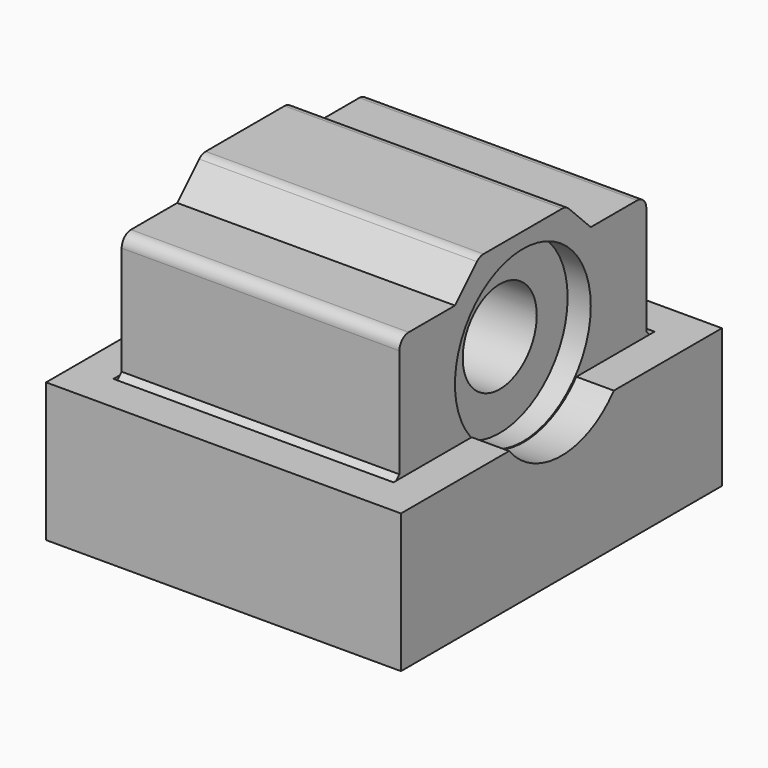
from build123d import *

# Parameters (mm, degrees)
F1_R              = 11
F2_DEPTH          = 18
F1_R_2            = 6
F3_DEPTH          = 15
F4_SIZE           = 0.99999
F5_R              = 1.5
F6_W              = 46
F6_H              = 52
F6_W_2            = 36.3
F6_H_2            = 42.3
F6_W_3            = 26
F6_H_3            = 23.35
F6_H_4            = 7.15
F7_DEPTH          = 10
F8_DEPTH          = 8
F10_D             = 5.5
F10_DEPTH         = 20
F10_CBORE_D       = 9.75
F10_CBORE_DEPTH   = 5
F10_TIP           = 1.6523667023
F10_2_D           = 5.5
F10_2_DEPTH       = 20
F10_2_CBORE_D     = 9.75
F10_2_CBORE_DEPTH = 5
F10_2_TIP         = 1.6523667023
F11_DEPTH         = 57.8


# Not quite as in the source:
# - a fillet or chamfer is up to 0.001 mm smaller than in the source, because OpenCascade refuses the exact size


with BuildPart() as f2:
    # F1 (on Right) → F2 (new body, symmetric)
    with BuildSketch(Plane.YZ):
        Polygon((-7.5, 0), (0, 0), (7.5, 0), (7.5, -1), (21, -1), (21, 6.4), (20, 6.4), (20, 23), (11, 23), (7, 27), (0, 27), (-7, 27), (-11, 23), (-20, 23), (-20, 6.4), (-21, 6.4), (-21, -1), (-7.5, -1), align=None)
        with Locations((0, 14)):
            Circle(F1_R, mode=Mode.SUBTRACT)
    extrude(amount=F2_DEPTH, both=True)

    # F4 (size 1 in the source; OpenCascade refuses exactly that, so slightly less here)
    f4_edges = [f2.edges().sort_by_distance(p)[0] for p in [
        (0, -20, 6.4),
        (0, 20, 6.4),
        (0, -7.5, 0),
        (0, 7.5, 0),
    ]]
    chamfer(f4_edges, length=F4_SIZE)

    # F5
    f5_edges = [f2.edges().sort_by_distance(p)[0] for p in [
        (0, -7, 27),
        (0, 7, 27),
        (0, -20, 23),
        (0, 20, 23),
    ]]
    fillet(f5_edges, radius=F5_R)

    # F10
    with Locations(Plane(origin=(0, 0, -11), x_dir=(1, 0, 0), z_dir=(0, 0, -1))):
        with Locations((-13, -15.85), (13, -15.85), (-13, 14.65), (13, 14.65)):
            CounterBoreHole(F10_D / 2, F10_CBORE_D / 2, F10_CBORE_DEPTH, depth=F10_DEPTH)
            with Locations((0, 0, -(F10_DEPTH + F10_TIP / 2))):  # 118° drill point
                Cone(0, F10_D / 2, F10_TIP, mode=Mode.SUBTRACT)


with BuildPart() as f3:
    # F1 (on Right) → F3 (new body, symmetric)
    with BuildSketch(Plane.YZ):
        with Locations((0, 14)):
            Circle(F1_R)
        with Locations((0, 14)):
            Circle(F1_R_2, mode=Mode.SUBTRACT)
    extrude(amount=F3_DEPTH, both=True)


with BuildPart() as f7:
    # F6 (on face) → F7 (new body)
    with BuildSketch(Plane(origin=(0, 0, -1), x_dir=(1, 0, 0), z_dir=(0, 0, -1))):
        Rectangle(F6_W, F6_H)
        Rectangle(F6_W_2, F6_H_2, mode=Mode.SUBTRACT)
        Rectangle(F6_W_2, F6_H_2)
        Polygon((18, 21), (18, 7.5), (18, -21), (-18, -21), (-18, 7.5), (-18, 21), align=None, mode=Mode.SUBTRACT)
        with Locations((0, -4.175)):
            Rectangle(F6_W_3, F6_H_3)
        Polygon((18, 7.5), (13, 7.5), (13, -15.85), (-13, -15.85), (-13, 7.5), (-18, 7.5), (-18, -21), (18, -21), align=None)
        Polygon((-13, 14.65), (13, 14.65), (13, 7.5), (18, 7.5), (18, 21), (-18, 21), (-18, 7.5), (-13, 7.5), align=None)
        with Locations((0, 11.075)):
            Rectangle(F6_W_3, F6_H_4)
    extrude(amount=F7_DEPTH)

    # F6 (on face) → F8 (join)
    with BuildSketch(Plane(origin=(0, 0, -1), x_dir=(1, 0, 0), z_dir=(0, 0, -1))):
        Rectangle(F6_W, F6_H)
        Rectangle(F6_W_2, F6_H_2, mode=Mode.SUBTRACT)
    extrude(amount=-F8_DEPTH)

    # F10#2
    with Locations(Plane(origin=(0, 0, -11), x_dir=(1, 0, 0), z_dir=(0, 0, -1))):
        with Locations((-13, -15.85), (13, -15.85), (-13, 14.65), (13, 14.65)):
            CounterBoreHole(F10_2_D / 2, F10_2_CBORE_D / 2, F10_2_CBORE_DEPTH, depth=F10_2_DEPTH)
            with Locations((0, 0, -(F10_2_DEPTH + F10_2_TIP / 2))):  # 118° drill point
                Cone(0, F10_2_D / 2, F10_2_TIP, mode=Mode.SUBTRACT)

    # F1 (on Right) → F11 (cut, symmetric)
    with BuildSketch(Plane.YZ):
        with Locations((0, 14)):
            Circle(F1_R)
        with Locations((0, 14)):
            Circle(F1_R_2, mode=Mode.SUBTRACT)
        with Locations((0, 14)):
            Circle(F1_R_2)
    extrude(amount=F11_DEPTH, both=True, mode=Mode.SUBTRACT)


solid = Compound([f2.part, f3.part, f7.part])
